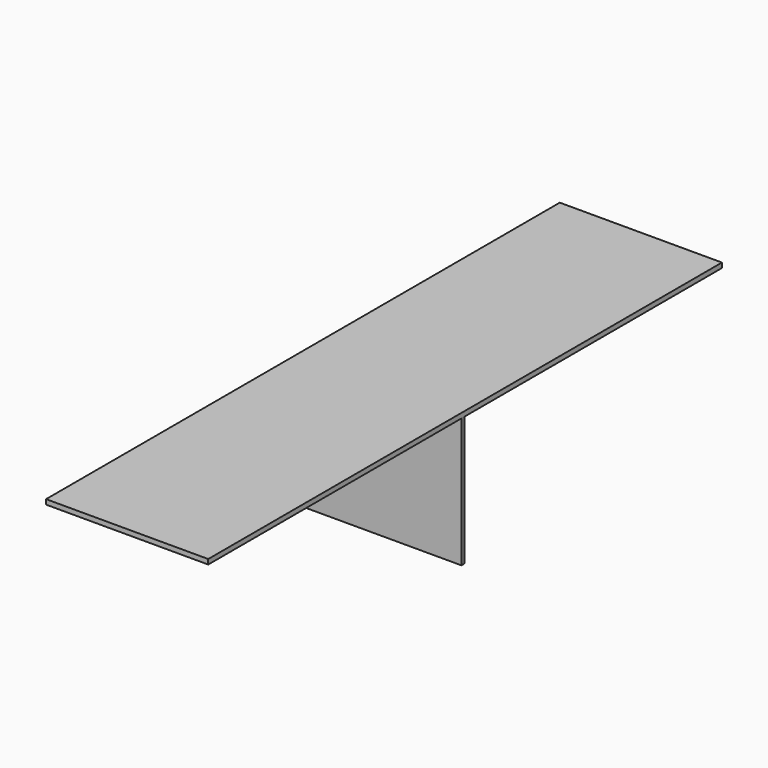
from build123d import *

# Parameters (mm, degrees)
F3_DEPTH = 30
F1_W     = 1000
F1_H     = 800
F4_DEPTH = 25


# Not quite as in the source:
# - the program builds the solid bodies; features that only make, move or delete a surface that nothing else refers to are left out


with BuildPart() as f3:
    # F0 (on Top) → F3 (new body)
    with BuildSketch(Plane.XY):
        Polygon((500, 0), (500, 500), (-24.3693755725, 500), align=None)
        Polygon((-24.3693755725, 500), (500, 500), (500, 1250), (-211.1726416889, 1250), (-500, 953.5263180733), align=None)
        Polygon((500, 0), (-24.3693755725, 500), (-500, 500), (-500, -500), (-71.4285714286, -500), align=None)
        Polygon((-500, 500), (-24.3693755725, 500), (-500, 953.5263180733), align=None)
        Polygon((500, -500), (500, 0), (-71.4285714286, -500), align=None)
        Polygon((-211.1726416889, 1250), (500, 1250), (500, 1980), align=None)
        Polygon((-500, 1250), (-500, 953.5263180733), (-211.1726416889, 1250), align=None)
        Polygon((500, -1250), (500, -500), (-71.4285714286, -500), (-500, -875), (-160.6334841629, -1250), align=None)
        Polygon((-500, -875), (-71.4285714286, -500), (-500, -500), align=None)
        Polygon((-500, 1250), (-211.1726416889, 1250), (500, 1980), (-500, 1980), align=None)
        Polygon((500, -1980), (500, -1250), (-160.6334841629, -1250), align=None)
        Polygon((-160.6334841629, -1250), (-500, -875), (-500, -1250), align=None)
        Polygon((500, -1980), (-160.6334841629, -1250), (-500, -1250), (-500, -1980), align=None)
    extrude(amount=F3_DEPTH)

    # F1 (on Front) → F4 (join)
    with BuildSketch(Plane.XZ):
        with Locations((-2.6259482768, -400)):
            Rectangle(F1_W, F1_H)
    extrude(amount=F4_DEPTH)


solid = f3.part
